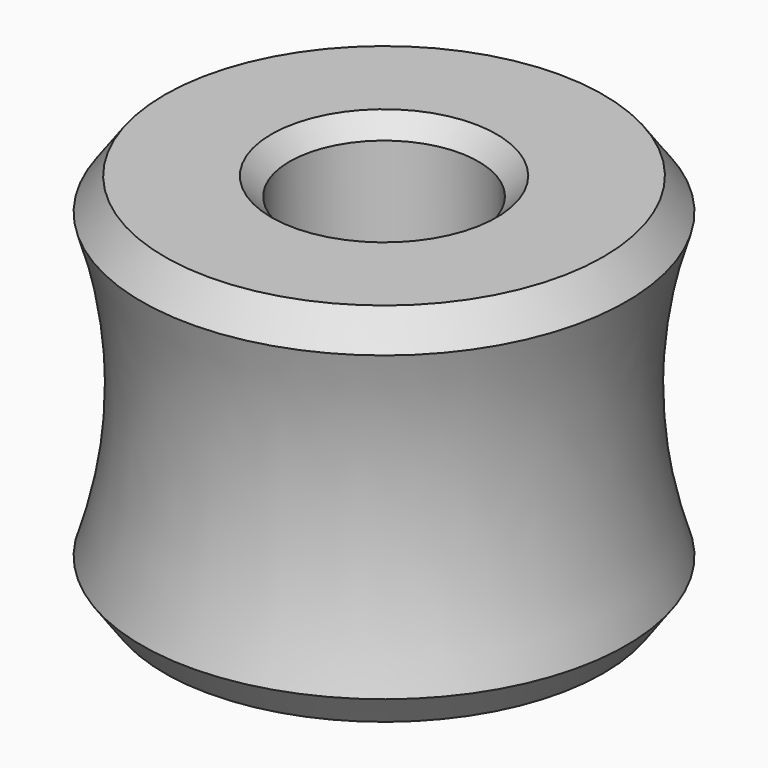
from build123d import *

# Parameters (mm, degrees)
F2_SIZE = 1


# Not quite as in the source:
# - a fillet or chamfer that OpenCascade refuses, or shapes differently, is made with other operations: its cross-section is extruded or revolved along the edge and cut away or added


with BuildPart() as f1:
    # F0 (on Front) → F1 (revolve)
    with BuildSketch(Plane.XZ):
        with BuildLine():
            Line((-5.2, 0), (-5.2, 20.18))
            Line((-5.2, 20.18), (-14, 20.18))
            ThreePointArc((-14, 20.18), (-12, 10.09), (-14, 0))
            Line((-14, 0), (-5.2, 0))
        make_face()
    revolve(axis=Axis((0, 0, 10.09), (0, 0, 1)))

    # F2
    f2_edges = [f1.edges().sort_by_distance(p)[0] for p in [
        (5.2, 0, 0),
        (5.2, 0, 20.18),
        (-5.2, 0, 10.09),
    ]]
    chamfer(f2_edges, length=F2_SIZE)

    # F3: chamfer of 2 on 3 edges, made by hand

    # F3_s1 → F3_t2 (revolve, cut)
    with BuildSketch(Plane.XZ):
        with BuildLine():
            Line((-13.3927401151, 18.3553817289), (-12.0288953822, 20.2448671044))
            Line((-12.0288953822, 20.2448671044), (-12.0288953822, 20.2848671044))
            ThreePointArc((-12.0288953822, 20.2848671044), (-13.0144476911, 20.22), (-14, 20.22))
            Line((-14, 20.22), (-14.0369756569, 20.1647421889))
            ThreePointArc((-14.0369756569, 20.1647421889), (-13.6870919943, 19.2711305309), (-13.4307048554, 18.3427849635))
            Line((-13.4307048554, 18.3427849635), (-13.3927401151, 18.3553817289))
        make_face()
    revolve(axis=Axis((0, 0, 20.18), (0, 0, 1)), mode=Mode.SUBTRACT)

    # F3_s3 → F3_t4 (revolve, cut)
    with BuildSketch(Plane.XZ):
        with BuildLine():
            Line((-12.0288953822, -0.0648671044), (-13.3927401151, 1.8246182711))
            Line((-13.3927401151, 1.8246182711), (-13.4307048554, 1.8372150365))
            ThreePointArc((-13.4307048554, 1.8372150365), (-13.6870919943, 0.9088694691), (-14.0369756569, 0.0152578111))
            Line((-14.0369756569, 0.0152578111), (-14, -0.04))
            ThreePointArc((-14, -0.04), (-13.0144476911, -0.04), (-12.0288953822, -0.1048671044))
            Line((-12.0288953822, -0.1048671044), (-12.0288953822, -0.0648671044))
        make_face()
    revolve(axis=Axis((0, 0, 0), (0, 0, 1)), mode=Mode.SUBTRACT)


solid = f1.part
